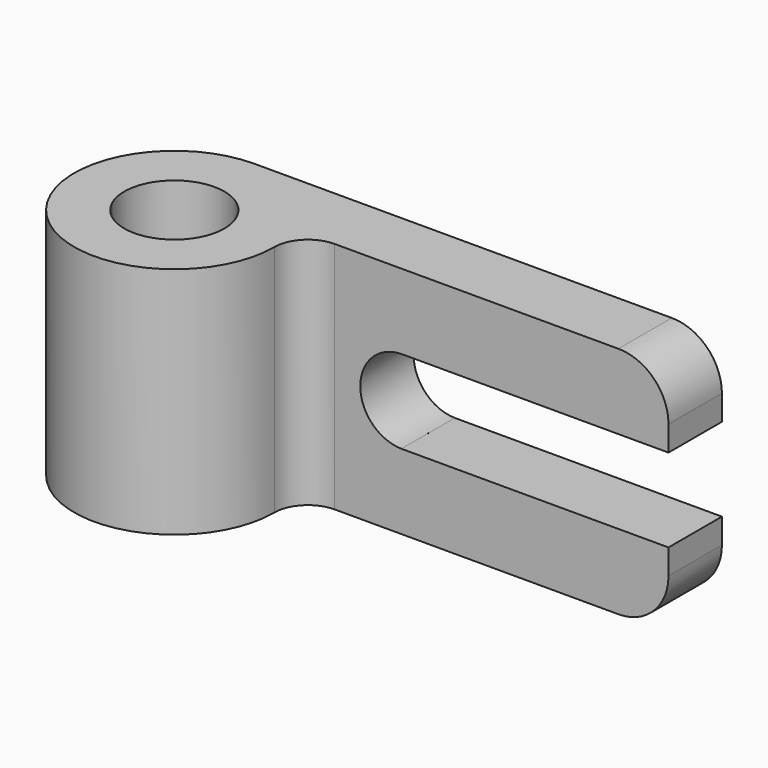
from build123d import *

# Parameters (mm, degrees)
F0_R        = 9.525
F1_DEPTH    = 44.45
F2_W        = 50.8
F2_H        = 15.875
F4_DEPTH    = 12.7
F5_R        = 9.525
F6_T1_DEPTH = 44.45


# Not quite as in the source:
# - a fillet or chamfer that OpenCascade refuses, or shapes differently, is made with other operations: its cross-section is extruded or revolved along the edge and cut away or added
# - a length typed as a fraction of an inch, garbled in the dataset ("3 / 203.2 mm" for 3/8 in), is restored


with BuildPart() as f1:
    # F0 (on Top) → F1 (new body)
    with BuildSketch(Plane.XY):
        with BuildLine():
            ThreePointArc((0, 19.05), (-13.4703841816, -13.4703841816), (19.05, 0))
            ThreePointArc((19.05, 0), (18.7756525614, 3.2213926947), (17.9605122421, 6.35))
            ThreePointArc((17.9605122421, 6.35), (10.9985226281, 15.5542598667), (0, 19.05))
        make_face()
        Circle(F0_R, mode=Mode.SUBTRACT)
        with BuildLine():
            ThreePointArc((0, 19.05), (10.9985226281, 15.5542598667), (17.9605122421, 6.35))
            Line((17.9605122421, 6.35), (88.9, 6.35))
            Line((88.9, 6.35), (88.9, 19.05))
            Line((88.9, 19.05), (0, 19.05))
        make_face()
    extrude(amount=F1_DEPTH)

    # F3 (on face) + F2 (on face) → F4 (cut)
    with BuildSketch(Plane.XZ.offset(-6.35)):
        with BuildLine():
            Line((38.1, 14.2883619165), (38.1, 30.1616380835))
            ThreePointArc((38.1, 30.1616380835), (30.279470861, 22.225), (38.1, 14.2883619165))
        make_face()
    with BuildSketch(Plane.XZ.offset(-6.35)):
        with Locations((63.5, 22.225)):
            Rectangle(F2_W, F2_H)
    extrude(amount=-F4_DEPTH, mode=Mode.SUBTRACT)

    # F5
    f5_edges = [f1.edges().sort_by_distance(p)[0] for p in [
        (88.9, 12.7, 44.45),
        (88.9, 12.7, 0),
    ]]
    fillet(f5_edges, radius=F5_R)

    # F6: fillet of radius 6.35 on 1 edges, made by hand

    # F6_s2 → F6_t1 (join)
    with BuildSketch(Plane.XY):
        with BuildLine():
            ThreePointArc((19.05, 0), (20.9098719395, 4.4901280605), (25.4, 6.35))
            Line((25.4, 6.35), (17.9605122421, 6.35))
            ThreePointArc((17.9605122421, 6.35), (18.7756525614, 3.2213926947), (19.05, 0))
        make_face()
    extrude(amount=F6_T1_DEPTH)


solid = f1.part
